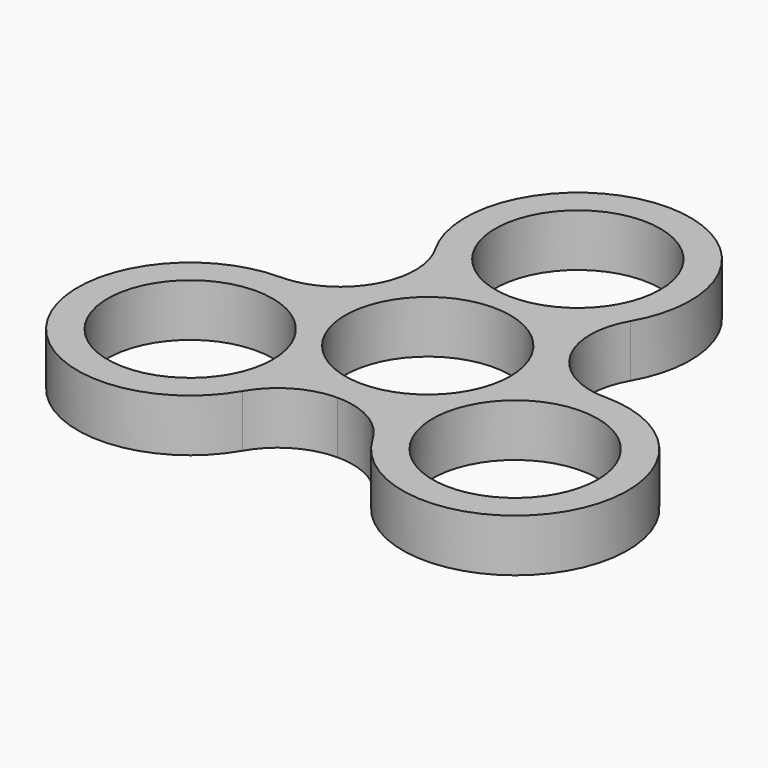
from build123d import *

# Parameters (mm, degrees)
F0_R     = 11
F1_DEPTH = 7
F2_R     = 9.999


# Not quite as in the source:
# - a fillet or chamfer is up to 0.001 mm smaller than in the source, because OpenCascade refuses the exact size


with BuildPart() as f1:
    # F0 (on Top) → F1 (new body)
    with BuildSketch(Plane.XY):
        with BuildLine():
            ThreePointArc((8.2915619759, 12.5), (0, 40), (-8.2915619759, 12.5))
            ThreePointArc((-8.2915619759, 12.5), (-12.9903810568, 7.5), (-14.9710985352, 0.9307033082))
            ThreePointArc((-14.9710985352, 0.9307033082), (-34.6410161514, -20), (-6.6795365594, -13.4307033082))
            ThreePointArc((-6.6795365594, -13.4307033082), (0, -15), (6.6795365594, -13.4307033082))
            ThreePointArc((6.6795365594, -13.4307033082), (34.6410161514, -20), (14.9710985352, 0.9307033082))
            ThreePointArc((14.9710985352, 0.9307033082), (12.9903810568, 7.5), (8.2915619759, 12.5))
        make_face()
        with Locations((-21.6506350946, -12.5)):
            Circle(F0_R, mode=Mode.SUBTRACT)
        with Locations((21.6506350946, -12.5)):
            Circle(F0_R, mode=Mode.SUBTRACT)
        Circle(F0_R, mode=Mode.SUBTRACT)
        with Locations((0, 25)):
            Circle(F0_R, mode=Mode.SUBTRACT)
    extrude(amount=F1_DEPTH)

    # F2 (radius 10 in the source; OpenCascade refuses exactly that, so slightly less here)
    f2_edges = [f1.edges().sort_by_distance(p)[0] for p in [
        (-8.291562, 12.5, 3.5),
        (-14.971099, 0.930703, 3.5),
        (-6.679537, -13.430703, 3.5),
        (6.679537, -13.430703, 3.5),
        (14.971099, 0.930703, 3.5),
        (8.291562, 12.5, 3.5),
    ]]
    fillet(f2_edges, radius=F2_R)


solid = f1.part
